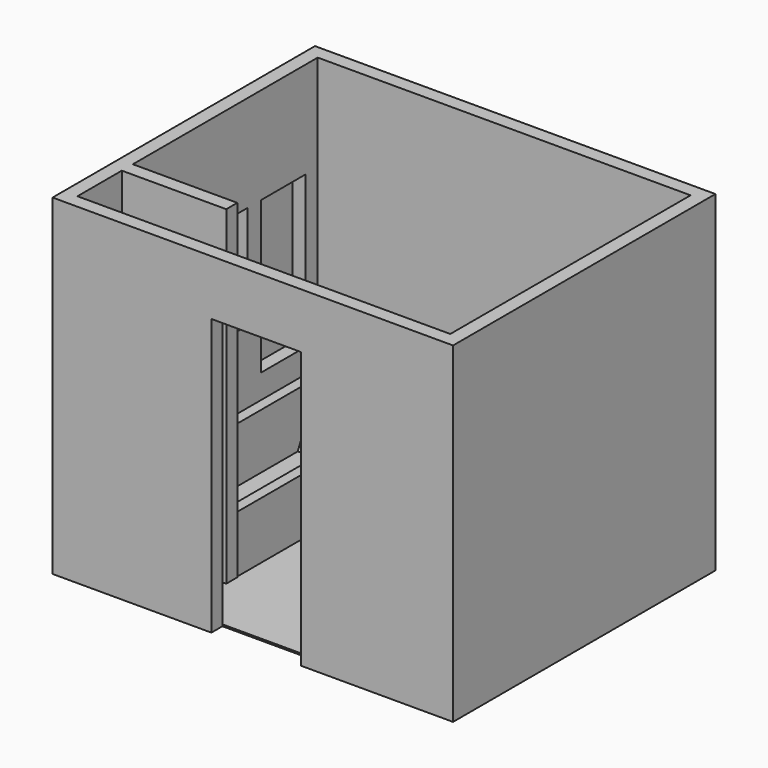
from build123d import *

# Parameters (mm, degrees)
F0_W      = 2946.4
F0_H      = 2413
F1_DEPTH  = 2438.4
F2_W      = 2743.2
F2_H      = 2209.8
F3_DEPTH  = 2425.7
F4_W      = 762
F4_H      = 1700.022
F5_DEPTH  = 431.8
F6_W      = 609.6
F6_H      = 1547.622
F7_DEPTH  = 406.4
F8_SIZE2  = 203.19999
F8_SIZE   = 406.39999
F9_W      = 768.35
F9_H      = 101.6
F10_DEPTH = 2438.4
F11_W     = 660.4
F11_H     = 2032
F12_DEPTH = 101.6
F13_W     = 406.4
F13_H     = 1117.6
F13_H_2   = 762
F13_H_3   = 457.2
F14_DEPTH = 95.25


# Not quite as in the source:
# - a fillet or chamfer is up to 0.001 mm smaller than in the source, because OpenCascade refuses the exact size


with BuildPart() as f1:
    # F0 (on Top) → F1 (new body)
    with BuildSketch(Plane.XY):
        Rectangle(F0_W, F0_H)
    extrude(amount=F1_DEPTH)

    # F2 (on face) → F3 (cut)
    with BuildSketch(Plane.XY.offset(2438.4)):
        Rectangle(F2_W, F2_H)
    extrude(amount=-F3_DEPTH, mode=Mode.SUBTRACT)

    # F9 (on Top) → F10 (join)
    with BuildSketch(Plane.XY):
        with Locations((-987.425, -645.922)):
            Rectangle(F9_W, F9_H)
    extrude(amount=F10_DEPTH)

    # F11 (on face) → F12 (cut)
    with BuildSketch(Plane.XZ.offset(1206.5)):
        with Locations((25.4, 1016)):
            Rectangle(F11_W, F11_H)
    extrude(amount=-F12_DEPTH, mode=Mode.SUBTRACT)

    # F13 (on face) → F14 (cut)
    with BuildSketch(Plane.YZ.offset(-1371.6)):
        with Locations((787.4, 1168.4)):
            Rectangle(F13_W, F13_H)
        with Locations((254, 1346.2)):
            Rectangle(F13_W, F13_H_2)
        with Locations((-279.4, 1498.6)):
            Rectangle(F13_W, F13_H_3)
    extrude(amount=-F14_DEPTH, mode=Mode.SUBTRACT)


with BuildPart() as f5:
    # F4 (on Top) → F5 (new body)
    with BuildSketch(Plane.XY):
        with Locations((-990.6, 254.889)):
            Rectangle(F4_W, F4_H)
    extrude(amount=F5_DEPTH)

    # F6 (on face) → F7 (cut)
    with BuildSketch(Plane.XY.offset(431.8)):
        with Locations((-990.6, 254.889)):
            Rectangle(F6_W, F6_H)
    extrude(amount=-F7_DEPTH, mode=Mode.SUBTRACT)

    # F8 (size 406.4 and 203.2 in the source; OpenCascade refuses exactly that, so slightly less here)
    f8_edges = [f5.edges().sort_by_distance(p)[0] for p in [
        (-990.6, 1028.7, 25.4),
        (-990.6, -518.922, 25.4),
    ]]
    chamfer(f8_edges, length=F8_SIZE, length2=F8_SIZE2)


solid = Compound([f1.part, f5.part])
